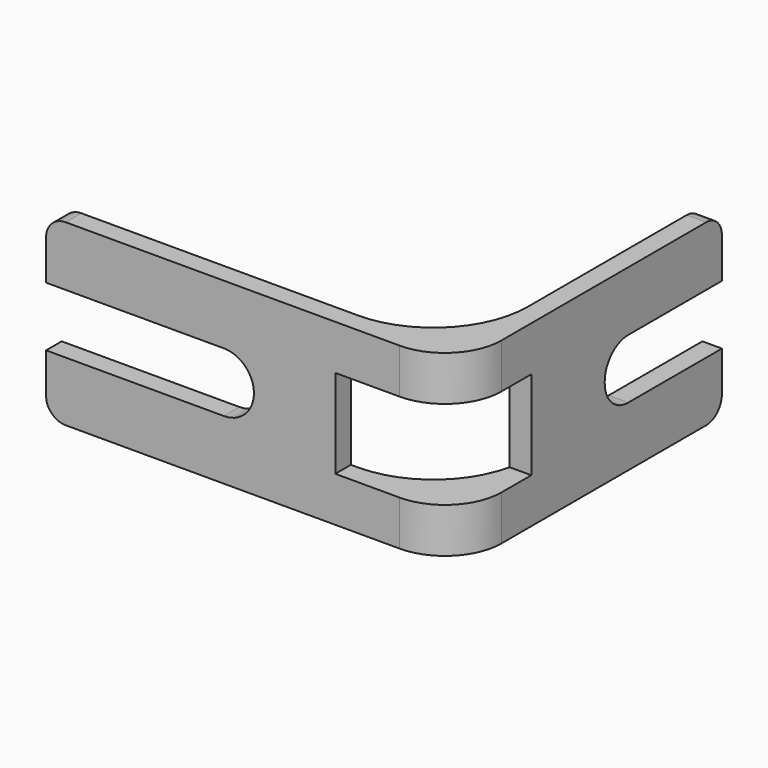
from build123d import *

# Parameters (mm, degrees)
F1_DEPTH     = 18.3
F2_W         = 17.3
F2_H         = 6.1
F3_DEPTH     = 25
F4_R         = 9.6568542495
F5_R         = 5.7941125497
F6_W         = 15
F6_H         = 6.1
F7_DEPTH     = 25
F8_R         = 3
F9_R         = 2
F11_DEPTH    = 7.6
F12_W        = 3.9829482868
F12_H        = 6.1
F13_DEPTH    = 25
F14_T1_DEPTH = 2
F15_DEPTH    = 1
F16_DEPTH    = 1
F17_DEPTH    = 2
F18_DEPTH    = 2
F19_DEPTH    = 0.5
F20_DEPTH    = 0.5


# Not quite as in the source:
# - a fillet or chamfer that OpenCascade refuses, or shapes differently, is made with other operations: its cross-section is extruded or revolved along the edge and cut away or added


with BuildPart() as f1:
    # F0 (on Top) → F1 (new body)
    with BuildSketch(Plane.XY):
        Polygon((4.2331174448, -18.8899510824), (-35.7668825552, -18.8899510824), (-35.7668825552, -20.8899510824), (6.2331174448, -20.8899510824), (6.2331174448, 13.1100489176), (4.2331174448, 13.1100489176), align=None)
    extrude(amount=F1_DEPTH)

    # F2 (on face) → F3 (cut)
    with BuildSketch(Plane(origin=(0, -18.8899510824, 0), x_dir=(-1, 0, 0), z_dir=(0, 1, 0))):
        with Locations((27.1168825552, 9.15)):
            Rectangle(F2_W, F2_H)
    extrude(amount=-F3_DEPTH, mode=Mode.SUBTRACT)

    # F4
    f4_edges = [f1.edges().sort_by_distance(p)[0] for p in [
        (4.233117, -18.889951, 9.15),
    ]]
    fillet(f4_edges, radius=F4_R)

    # F5
    f5_edges = [f1.edges().sort_by_distance(p)[0] for p in [
        (6.233117, -20.889951, 9.15),
    ]]
    fillet(f5_edges, radius=F5_R)

    # F6 (on face) → F7 (cut)
    with BuildSketch(Plane(origin=(4.2331174448, 0, 0), x_dir=(0, -1, 0), z_dir=(-1, 0, 0))):
        with Locations((-5.6100489176, 9.15)):
            Rectangle(F6_W, F6_H)
    extrude(amount=-F7_DEPTH, mode=Mode.SUBTRACT)

    # F8
    f8_edges = [f1.edges().sort_by_distance(p)[0] for p in [
        (5.233117, -1.889951, 6.1),
        (5.233117, -1.889951, 12.2),
    ]]
    fillet(f8_edges, radius=F8_R)

    # F9
    f9_edges = [f1.edges().sort_by_distance(p)[0] for p in [
        (5.233117, 13.110049, 0),
        (5.233117, 13.110049, 18.3),
        (-35.766883, -19.889951, 0),
        (-35.766883, -19.889951, 18.3),
    ]]
    fillet(f9_edges, radius=F9_R)

    # F10 (on face) → F11 (cut)
    with BuildSketch(Plane.XZ.offset(20.8899510824)):
        Polygon((7.5907320715, 6.1), (7.5907320715, 9.2), (7.5907320715, 12.2), (-4.1556255892, 12.2), (-4.1556255892, 6.1), align=None)
    extrude(amount=-F11_DEPTH, mode=Mode.SUBTRACT)

    # F12 (on face) → F13 (cut)
    with BuildSketch(Plane(origin=(0, -18.8899510824, 0), x_dir=(-1, 0, 0), z_dir=(0, 1, 0))):
        with Locations((16.4754084118, 9.15)):
            Rectangle(F12_W, F12_H)
    extrude(amount=-F13_DEPTH, mode=Mode.SUBTRACT)

    # F14: fillet of radius 3.0660512242 on 2 edges, made by hand

    # F14_s2 → F14_t1 (join)
    with BuildSketch(Plane.XZ.offset(18.8899510824)):
        with BuildLine():
            ThreePointArc((-14.4839342684, 9.1660512242), (-15.3819598805, 6.9980256121), (-17.5499854926, 6.1))
            Line((-17.5499854926, 6.1), (-14.4839342684, 6.1))
            Line((-14.4839342684, 6.1), (-14.4839342684, 9.1660512242))
        make_face()
        with BuildLine():
            ThreePointArc((-17.5499854926, 12.2), (-15.3819598805, 11.3019743879), (-14.4839342684, 9.1339487758))
            Line((-14.4839342684, 9.1339487758), (-14.4839342684, 12.2))
            Line((-14.4839342684, 12.2), (-17.5499854926, 12.2))
        make_face()
    extrude(amount=F14_T1_DEPTH)

    # F15 (cut): faces of the model
    f15_faces = [f1.faces().sort_by_distance(p)[0] for p in [
        (1.8734055755, -17.7191060476, 6.1),
        (1.8734055755, -17.7191060476, 12.2),
    ]]
    extrude(f15_faces, amount=-F15_DEPTH, dir=(0, 0, 1), mode=Mode.SUBTRACT)

    # F16 (cut): a face of the model
    f16_faces = [f1.faces().sort_by_distance(p)[0] for p in [
        (1.8734055755, -17.7191060476, 12.2),
    ]]
    extrude(f16_faces, amount=-F16_DEPTH, mode=Mode.SUBTRACT)

    # F17 (cut): a face of the model
    f17_faces = [f1.faces().sort_by_distance(p)[0] for p in [
        (-4.1556255892, -19.8481388351, 9.15),
    ]]
    extrude(f17_faces, amount=-F17_DEPTH, mode=Mode.SUBTRACT)

    # F18 (cut): a face of the model
    f18_faces = [f1.faces().sort_by_distance(p)[0] for p in [
        (4.7863785676, -13.2899510824, 9.15),
    ]]
    extrude(f18_faces, amount=-F18_DEPTH, mode=Mode.SUBTRACT)

    # F19 (cut): a face of the model
    f19_faces = [f1.faces().sort_by_distance(p)[0] for p in [
        (1.6308493787, -17.3698716383, 13.2),
    ]]
    extrude(f19_faces, amount=-F19_DEPTH, mode=Mode.SUBTRACT)

    # F20 (cut): a face of the model
    f20_faces = [f1.faces().sort_by_distance(p)[0] for p in [
        (1.6308493787, -17.3698716383, 5.1),
    ]]
    extrude(f20_faces, amount=-F20_DEPTH, mode=Mode.SUBTRACT)


solid = f1.part
